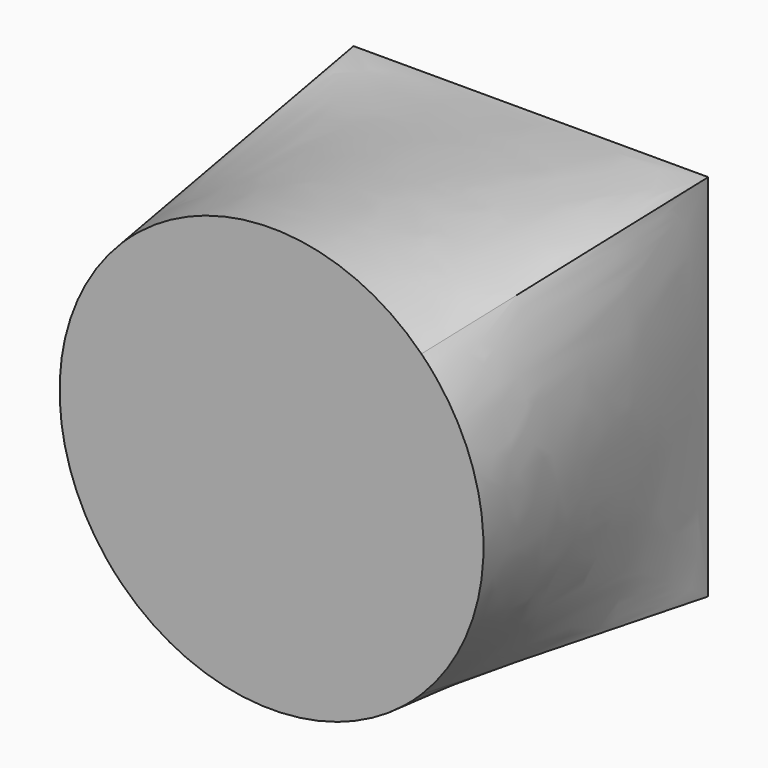
from build123d import *

# Parameters (mm, degrees)
F0_W = 54.9789518118
F0_H = 57.2138559073


# Not quite as in the source:
# - the arcs of a loft's sections are written as splines that run evenly, so that the points pair up as in the source's solid


with BuildPart() as f3:
    # F0 (on Front) → F3 section 0
    with BuildSketch(Plane.XZ):
        with Locations((-0.4469808191, -0.6704749539)):
            Rectangle(F0_W, F0_H)
    # F2 (on offset) → F3 section 1
    with BuildSketch(Plane.XZ.offset(50.8)):
        with BuildLine():
            add(Edge.make_bspline(
                [(-23.2313098206, 23.2313067227), (-24.75179529, 21.7108210505), (-26.1224920978, 20.0406219306), (-28.511767554, 16.4648179982), (-29.5302871228, 14.5593016045), (-31.1760485804, 10.5860812238), (-31.8032497745, 8.5184754826), (-32.6422515437, 4.3005272847), (-32.8540313728, 2.1502891251), (-32.8540310861, -2.1502935062), (-32.6422509702, -4.3005316375), (-31.8032486386, -8.5184797235), (-31.1760471688, -10.5860853811), (-29.5302851814, -14.5593055423), (-28.5117653584, -16.4648218002), (-26.1224894254, -20.040625414), (-24.7517923949, -21.7108243511), (-23.2313067227, -23.2313098206)],
                knots=[0, 0, 0, 0, 0.125, 0.125, 0.25, 0.25, 0.375, 0.375, 0.5, 0.5, 0.625, 0.625, 0.75, 0.75, 0.875, 0.875, 1, 1, 1, 1], degree=3))
            add(Edge.make_bspline(
                [(-23.2313067227, -23.2313098206), (-21.7108210505, -24.75179529), (-20.0406219306, -26.1224920978), (-16.4648179982, -28.511767554), (-14.5593016045, -29.5302871228), (-10.5860812238, -31.1760485804), (-8.5184754826, -31.8032497745), (-4.3005272847, -32.6422515437), (-2.1502891251, -32.8540313728), (2.1502935062, -32.8540310861), (4.3005316375, -32.6422509702), (8.5184797235, -31.8032486386), (10.5860853811, -31.1760471688), (14.5593055423, -29.5302851814), (16.4648218002, -28.5117653584), (20.040625414, -26.1224894254), (21.7108243511, -24.7517923949), (23.2313098206, -23.2313067227)],
                knots=[0, 0, 0, 0, 0.125, 0.125, 0.25, 0.25, 0.375, 0.375, 0.5, 0.5, 0.625, 0.625, 0.75, 0.75, 0.875, 0.875, 1, 1, 1, 1], degree=3))
            add(Edge.make_bspline(
                [(23.2313098206, -23.2313067227), (24.75179529, -21.7108210505), (26.1224920978, -20.0406219306), (28.511767554, -16.4648179982), (29.5302871228, -14.5593016045), (31.1760485804, -10.5860812238), (31.8032497745, -8.5184754826), (32.6422515437, -4.3005272847), (32.8540313728, -2.1502891251), (32.8540310861, 2.1502935062), (32.6422509702, 4.3005316375), (31.8032486386, 8.5184797235), (31.1760471688, 10.5860853811), (29.5302851814, 14.5593055423), (28.5117653584, 16.4648218002), (26.1224894254, 20.040625414), (24.7517923949, 21.7108243511), (23.2313067227, 23.2313098206)],
                knots=[0, 0, 0, 0, 0.125, 0.125, 0.25, 0.25, 0.375, 0.375, 0.5, 0.5, 0.625, 0.625, 0.75, 0.75, 0.875, 0.875, 1, 1, 1, 1], degree=3))
            add(Edge.make_bspline(
                [(23.2313067227, 23.2313098206), (21.7108210505, 24.75179529), (20.0406219306, 26.1224920978), (16.4648179982, 28.511767554), (14.5593016045, 29.5302871228), (10.5860812238, 31.1760485804), (8.5184754826, 31.8032497745), (4.3005272847, 32.6422515437), (2.1502891251, 32.8540313728), (-2.1502935062, 32.8540310861), (-4.3005316375, 32.6422509702), (-8.5184797235, 31.8032486386), (-10.5860853811, 31.1760471688), (-14.5593055423, 29.5302851814), (-16.4648218002, 28.5117653584), (-20.040625414, 26.1224894254), (-21.7108243511, 24.7517923949), (-23.2313098206, 23.2313067227)],
                knots=[0, 0, 0, 0, 0.125, 0.125, 0.25, 0.25, 0.375, 0.375, 0.5, 0.5, 0.625, 0.625, 0.75, 0.75, 0.875, 0.875, 1, 1, 1, 1], degree=3))
        make_face()
    loft(ruled=True)


solid = f3.part
